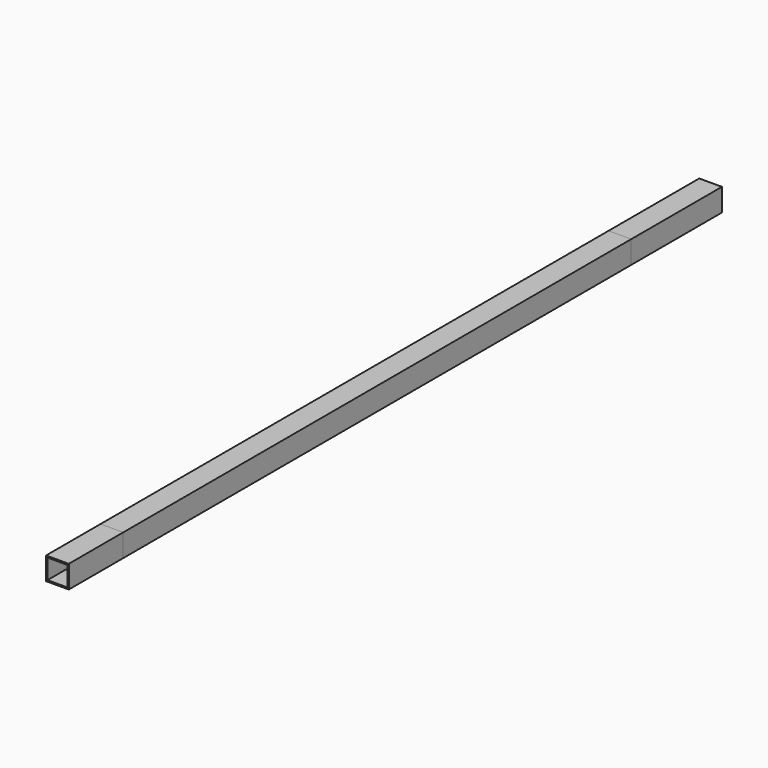
from build123d import *

# Parameters (mm, degrees)
F0_W      = 25.4
F0_H      = 25.4
F0_W_2    = 22.225
F0_H_2    = 22.225
F1_DEPTH  = 914.4
F2_DEPTH  = 279.4
F3_DEPTH  = 381
F4_DEPTH  = 381
F5_DEPTH  = 609.6
F6_DEPTH  = 838.2
F7_DEPTH  = 76.2
F8_DEPTH  = 838.2
F9_DEPTH  = 152.4
F11_DEPTH = 25.4
F13_DEPTH = 25.4
F14_DEPTH = 838.2
F15_DEPTH = 101.6
F16_DEPTH = 127


with BuildPart() as f1:
    # F0 (on Front) → F1 (new body)
    with BuildSketch(Plane.XZ):
        with Locations((12.7, 12.7)):
            Rectangle(F0_W, F0_H)
        with Locations((12.7, 12.7)):
            Rectangle(F0_W_2, F0_H_2, mode=Mode.SUBTRACT)
    extrude(amount=F1_DEPTH)


with BuildPart() as f2:
    # F0 (on Front) → F2 (new body)
    with BuildSketch(Plane.XZ):
        with Locations((12.7, 12.7)):
            Rectangle(F0_W, F0_H)
        with Locations((12.7, 12.7)):
            Rectangle(F0_W_2, F0_H_2, mode=Mode.SUBTRACT)
    extrude(amount=F2_DEPTH)


with BuildPart() as f3:
    # F0 (on Front) → F3 (new body)
    with BuildSketch(Plane.XZ):
        with Locations((12.7, 12.7)):
            Rectangle(F0_W, F0_H)
        with Locations((12.7, 12.7)):
            Rectangle(F0_W_2, F0_H_2, mode=Mode.SUBTRACT)
    extrude(amount=F3_DEPTH)


with BuildPart() as f4:
    # F0 (on Front) → F4 (new body)
    with BuildSketch(Plane.XZ):
        with Locations((12.7, 12.7)):
            Rectangle(F0_W, F0_H)
        with Locations((12.7, 12.7)):
            Rectangle(F0_W_2, F0_H_2, mode=Mode.SUBTRACT)
    extrude(amount=F4_DEPTH)


with BuildPart() as f5:
    # F0 (on Front) → F5 (new body)
    with BuildSketch(Plane.XZ):
        with Locations((12.7, 12.7)):
            Rectangle(F0_W, F0_H)
        with Locations((12.7, 12.7)):
            Rectangle(F0_W_2, F0_H_2, mode=Mode.SUBTRACT)
    extrude(amount=F5_DEPTH)


with BuildPart() as f6:
    # F0 (on Front) → F6 (new body)
    with BuildSketch(Plane.XZ):
        with Locations((12.7, 12.7)):
            Rectangle(F0_W, F0_H)
        with Locations((12.7, 12.7)):
            Rectangle(F0_W_2, F0_H_2, mode=Mode.SUBTRACT)
    extrude(amount=F6_DEPTH)


with BuildPart() as f7:
    # F0 (on Front) → F7 (new body)
    with BuildSketch(Plane.XZ):
        with Locations((12.7, 12.7)):
            Rectangle(F0_W, F0_H)
        with Locations((12.7, 12.7)):
            Rectangle(F0_W_2, F0_H_2, mode=Mode.SUBTRACT)
    extrude(amount=F7_DEPTH)


with BuildPart() as f8:
    # F0 (on Front) → F8 (new body)
    with BuildSketch(Plane.XZ):
        with Locations((12.7, 12.7)):
            Rectangle(F0_W, F0_H)
        with Locations((12.7, 12.7)):
            Rectangle(F0_W_2, F0_H_2, mode=Mode.SUBTRACT)
    extrude(amount=F8_DEPTH)

    # F12 (on face) → F13 (cut)
    with BuildSketch(Plane.YZ.offset(25.4)):
        Polygon((-25.4, 25.4), (0, 0), (0, 25.4), align=None)
        Polygon((-838.2, 25.4), (-838.2, 0), (-812.8, 25.4), align=None)
    extrude(amount=-F13_DEPTH, mode=Mode.SUBTRACT)


with BuildPart() as f9:
    # F0 (on Front) → F9 (new body)
    with BuildSketch(Plane.XZ):
        with Locations((12.7, 12.7)):
            Rectangle(F0_W, F0_H)
        with Locations((12.7, 12.7)):
            Rectangle(F0_W_2, F0_H_2, mode=Mode.SUBTRACT)
    extrude(amount=F9_DEPTH)

    # F10 (on face) → F11 (cut)
    with BuildSketch(Plane.YZ.offset(25.4)):
        Polygon((-152.4, 25.4), (-152.4, 0), (-127, 25.4), align=None)
        Polygon((-25.4, 25.4), (0, 0), (0, 25.4), align=None)
    extrude(amount=-F11_DEPTH, mode=Mode.SUBTRACT)


with BuildPart() as f14:
    # F0 (on Front) → F14 (new body)
    with BuildSketch(Plane.XZ):
        with Locations((12.7, 12.7)):
            Rectangle(F0_W, F0_H)
        with Locations((12.7, 12.7)):
            Rectangle(F0_W_2, F0_H_2, mode=Mode.SUBTRACT)
    extrude(amount=F14_DEPTH)


with BuildPart() as f15:
    # F0 (on Front) → F15 (new body)
    with BuildSketch(Plane.XZ):
        with Locations((12.7, 12.7)):
            Rectangle(F0_W, F0_H)
        with Locations((12.7, 12.7)):
            Rectangle(F0_W_2, F0_H_2, mode=Mode.SUBTRACT)
    extrude(amount=F15_DEPTH)


with BuildPart() as f16:
    # F0 (on Front) → F16 (new body)
    with BuildSketch(Plane.XZ):
        with Locations((12.7, 12.7)):
            Rectangle(F0_W, F0_H)
        with Locations((12.7, 12.7)):
            Rectangle(F0_W_2, F0_H_2, mode=Mode.SUBTRACT)
    extrude(amount=F16_DEPTH)


solid = Compound([f1.part, f2.part, f3.part, f4.part, f5.part, f6.part, f7.part, f8.part, f9.part, f14.part, f15.part, f16.part])
